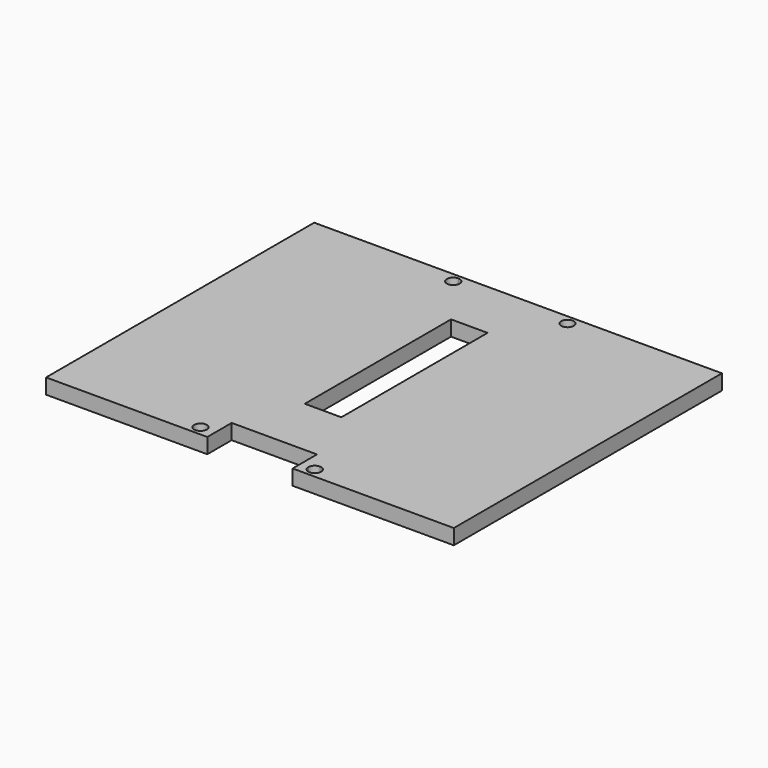
from build123d import *

# Parameters (mm, degrees)
F1_DEPTH = 3.175
F2_W     = 6.985
F2_H     = 3.175
F3_DEPTH = 6.35
F5_DEPTH = 25.4
F6_DEPTH = 25.4
F7_DEPTH = 26.6192
F8_DEPTH = 26.6192


# Not quite as in the source:
# - a feature names something its author has since deleted; it is built from what else it names


with BuildPart() as f1:
    # F0 (on Top) → F1 (new body)
    with BuildSketch(Plane.XY):
        Polygon((0, 63.5), (0, 0), (15.875, 0), (15.875, 12.7), (12.065, 12.7), (12.065, 50.8), (15.875, 50.8), (15.875, 63.5), align=None)
        Polygon((15.875, 12.7), (15.875, 0), (31.75, 0), (31.75, 63.5), (15.875, 63.5), (15.875, 50.8), (19.685, 50.8), (19.685, 12.7), align=None)
    extrude(amount=F1_DEPTH)

    # F2 (on face) → F3 (join)
    with BuildSketch(Plane.XZ):
        with Locations((3.4925, 1.5875)):
            Rectangle(F2_W, F2_H)
        with Locations((28.2575, 1.5875)):
            Rectangle(F2_W, F2_H)
    extrude(amount=F3_DEPTH)

    # F4 (on face) → F5 (cut)
    with BuildSketch(Plane.XY.offset(3.175)):
        with BuildLine():
            ThreePointArc((5.29375, -4.35), (3.0318335149, -3.4130835149), (3.96875, -5.675))
            Line((3.96875, -5.675), (3.96875, -4.35))
            Line((3.96875, -4.35), (5.29375, -4.35))
        make_face()
        with BuildLine():
            Line((3.96875, -4.35), (3.96875, -5.675))
            ThreePointArc((3.96875, -5.675), (4.9056664851, -5.2869164851), (5.29375, -4.35))
            Line((5.29375, -4.35), (3.96875, -4.35))
        make_face()
        with BuildLine():
            ThreePointArc((27.78125, -3.025), (26.8443335149, -3.4130835149), (26.45625, -4.35))
            Line((26.45625, -4.35), (27.78125, -4.35))
            Line((27.78125, -4.35), (27.78125, -3.025))
        make_face()
    extrude(amount=-F5_DEPTH, mode=Mode.SUBTRACT)

    # F4 (on face) → F6 (cut)
    with BuildSketch(Plane.XY.offset(3.175)):
        with BuildLine():
            ThreePointArc((29.10625, 61.5), (27.78125, 62.825), (26.45625, 61.5))
            ThreePointArc((26.45625, 61.5), (27.78125, 60.175), (29.10625, 61.5))
        make_face()
        with BuildLine():
            ThreePointArc((5.29375, 61.5), (4.9056664851, 62.4369164851), (3.96875, 62.825))
            ThreePointArc((3.96875, 62.825), (3.0318335149, 60.5630835149), (5.29375, 61.5))
        make_face()
        with BuildLine():
            Line((27.78125, -4.35), (26.45625, -4.35))
            ThreePointArc((26.45625, -4.35), (26.8443335149, -5.2869164851), (27.78125, -5.675))
            ThreePointArc((27.78125, -5.675), (28.7181664851, -5.2869164851), (29.10625, -4.35))
            ThreePointArc((29.10625, -4.35), (28.7181664851, -3.4130835149), (27.78125, -3.025))
            Line((27.78125, -3.025), (27.78125, -4.35))
        make_face()
    extrude(amount=-F6_DEPTH, mode=Mode.SUBTRACT)

    # F7 (add): a face of the model
    f7_faces = [f1.faces().sort_by_distance(p)[0] for p in [
        (31.75, 28.575, 1.5875),
    ]]
    extrude(f7_faces, amount=F7_DEPTH)

    # F8 (add): a face of the model
    f8_faces = [f1.faces().sort_by_distance(p)[0] for p in [
        (0, 28.575, 1.5875),
    ]]
    extrude(f8_faces, amount=F8_DEPTH)


solid = f1.part
